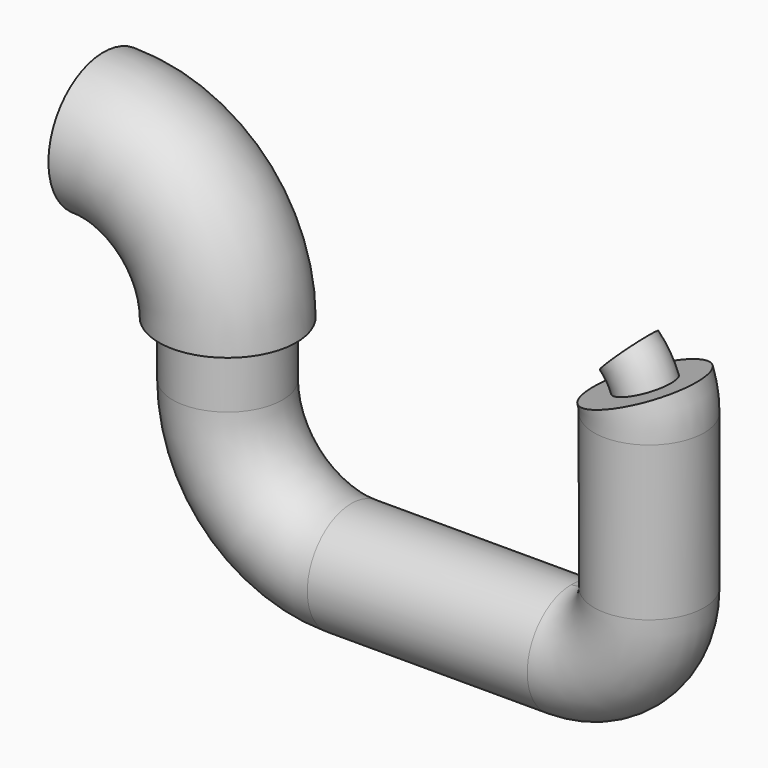
from build123d import *

# Parameters (mm, degrees)
F0_R      = 12.5
F2_ANGLE  = 90
F3_R      = 10
F4_DEPTH  = 10
F5_R      = 10
F8_ANGLE  = 90
F9_R      = 10
F10_DEPTH = 40
F12_ANGLE = 90
F13_R     = 10
F14_DEPTH = 28
F15_R     = 10
F15_R_2   = 5
F17_ANGLE = 20
F18_ANGLE = 45


# Not quite as in the source:
# - the program builds the solid bodies; features that only make, move or delete a surface that nothing else refers to are left out


with BuildPart() as f2:
    # F0 (on Right) → F2 (revolve)
    with BuildSketch(Plane.YZ):
        Circle(F0_R)
    revolve(axis=Axis((0, 8.0864932388, -22.5855782628), (0, 1, 0)), revolution_arc=F2_ANGLE)

    # F3 (on face) → F4 (join)
    with BuildSketch(Plane(origin=(0, 0, -22.5855782628), x_dir=(1, 0, 0), z_dir=(0, 0, -1))):
        with Locations((22.5855782628, 0)):
            Circle(F3_R)
    extrude(amount=F4_DEPTH)

    # F5 (on face) → F8 (revolve)
    with BuildSketch(Plane(origin=(0, 0, -32.5855782628), x_dir=(1, 0, 0), z_dir=(0, 0, -1))):
        with Locations((22.5855782628, 0)):
            Circle(F5_R)
    revolve(axis=Axis((45.0843572617, 2.1267626435, -32.5855782628), (0, -1, 0)), revolution_arc=F8_ANGLE)

    # F9 (on face) → F10 (join)
    with BuildSketch(Plane.YZ.offset(45.0843572617)):
        with Locations((0, -55.0843572617)):
            Circle(F9_R)
    extrude(amount=F10_DEPTH)

    # F11 (on face) → F12 (revolve)
    with BuildSketch(Plane.YZ.offset(85.0843572617)):
        with BuildLine():
            ThreePointArc((0, -45.0843572617), (-7.0710678119, -62.1554250735), (10, -55.0843572617))
            ThreePointArc((10, -55.0843572617), (7.0710678119, -48.0132894498), (0, -45.0843572617))
        make_face()
    revolve(axis=Axis((85.0843572617, 1.324259676, -40.921472013), (0, -1, 0)), revolution_arc=F12_ANGLE)

    # F13 (on face) → F14 (join)
    with BuildSketch(Plane.XY.offset(-40.921472013)):
        with Locations((99.2472425103, 0)):
            Circle(F13_R)
    extrude(amount=F14_DEPTH)

    # F15 (on face) → F17 (revolve)
    with BuildSketch(Plane.XY.offset(-12.921472013)):
        with Locations((99.2472425103, 0)):
            Circle(F15_R)
        with Locations((99.2472425103, 0)):
            Circle(F15_R_2, mode=Mode.SUBTRACT)
    revolve(axis=Axis((86.8095904589, -1.1897617951, -12.921472013), (0, -1, 0)), revolution_arc=F17_ANGLE)

    # F16 (on face) → F18 (revolve)
    with BuildSketch(Plane.XY.offset(-12.921472013)):
        with BuildLine():
            ThreePointArc((94.2472425103, 0), (99.2472425103, -5), (104.2472425103, 0))
            ThreePointArc((104.2472425103, 0), (99.2472425103, 5), (94.2472425103, 0))
        make_face()
    revolve(axis=Axis((86.8095904589, -1.1897617951, -12.921472013), (0, -1, 0)), revolution_arc=F18_ANGLE)


solid = f2.part
